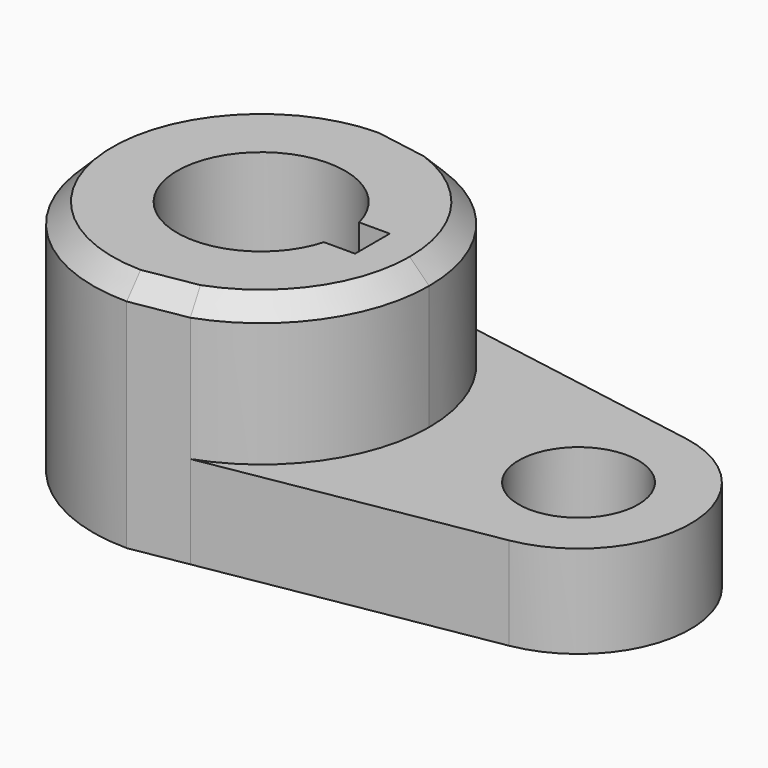
from build123d import *

# Parameters (mm, degrees)
F0_R       = 10.16
F1_DEPTH   = 40.2336
F2_R       = 10.16
F3_DEPTH   = 24.4602
F4_C1_SIZE = 3.302
F4_C2_SIZE = 3.302
F4_C3_SIZE = 3.302
F4_C4_SIZE = 3.302


with BuildPart() as f1:
    # F0 (on Top) → F1 (new body)
    with BuildSketch(Plane.XY):
        with BuildLine():
            Line((57.1919272622, 18.7764181619), (9.5121844836, 26.9452959039))
            ThreePointArc((9.5121844836, 26.9452959039), (23.3274655355, 16.5033322905), (28.575, 0))
            ThreePointArc((28.575, 0), (23.3274655355, -16.5033322905), (9.5121844836, -26.9452959039))
            Line((9.5121844836, -26.9452959039), (57.1919272622, -18.7764181619))
            ThreePointArc((57.1919272622, -18.7764181619), (73.025, 0), (57.1919272622, 18.7764181619))
        make_face()
        with Locations((53.975, 0)):
            Circle(F0_R, mode=Mode.SUBTRACT)
        with BuildLine():
            Line((9.5121844836, 26.9452959039), (0, 28.575))
            ThreePointArc((0, 28.575), (-28.575, 0), (0, -28.575))
            Line((0, -28.575), (9.5121844836, -26.9452959039))
            ThreePointArc((9.5121844836, -26.9452959039), (23.3274655355, -16.5033322905), (28.575, 0))
            ThreePointArc((28.575, 0), (23.3274655355, 16.5033322905), (9.5121844836, 26.9452959039))
        make_face()
        with BuildLine():
            ThreePointArc((13.7595011415, -3.8482183654), (-14.2865339733, 0.1661423458), (13.845272005, 3.5271942616))
            Line((13.845272005, 3.5271942616), (19.0572988585, 3.5271942616))
            Line((19.0572988585, 3.5271942616), (19.0572988585, -3.8482183654))
            Line((19.0572988585, -3.8482183654), (13.7595011415, -3.8482183654))
        make_face(mode=Mode.SUBTRACT)
    extrude(amount=F1_DEPTH)

    # F2 (on face) → F3 (cut)
    with BuildSketch(Plane.XY.offset(40.2336)):
        with BuildLine():
            Line((57.1919272622, 18.7764181619), (9.5121844836, 26.9452959039))
            ThreePointArc((9.5121844836, 26.9452959039), (23.3274655355, 16.5033322905), (28.575, 0))
            ThreePointArc((28.575, 0), (23.3274655355, -16.5033322905), (9.5121844836, -26.9452959039))
            Line((9.5121844836, -26.9452959039), (57.1919272622, -18.7764181619))
            ThreePointArc((57.1919272622, -18.7764181619), (73.025, 0), (57.1919272622, 18.7764181619))
        make_face()
        with Locations((53.975, 0)):
            Circle(F2_R, mode=Mode.SUBTRACT)
    extrude(amount=-F3_DEPTH, mode=Mode.SUBTRACT)

    # F4: chamfer of 3.302 on 4 edges, made by hand

    # F4_c1
    f4_c1_edges = [f1.edges().sort_by_distance(p)[0] for p in [
        (4.7560922418, 27.760147952, 40.2336),
    ]]
    chamfer(f4_c1_edges, length=F4_C1_SIZE)

    # F4_c2
    f4_c2_edges = [f1.edges().sort_by_distance(p)[0] for p in [
        (4.7560922418, -27.760147952, 40.2336),
    ]]
    chamfer(f4_c2_edges, length=F4_C2_SIZE)

    # F4_c3
    f4_c3_edges = [f1.edges().sort_by_distance(p)[0] for p in [
        (-28.575, 0, 40.2336),
    ]]
    chamfer(f4_c3_edges, length=F4_C3_SIZE)

    # F4_c4
    f4_c4_edges = [f1.edges().sort_by_distance(p)[0] for p in [
        (28.575, 0, 40.2336),
    ]]
    chamfer(f4_c4_edges, length=F4_C4_SIZE)


solid = f1.part
